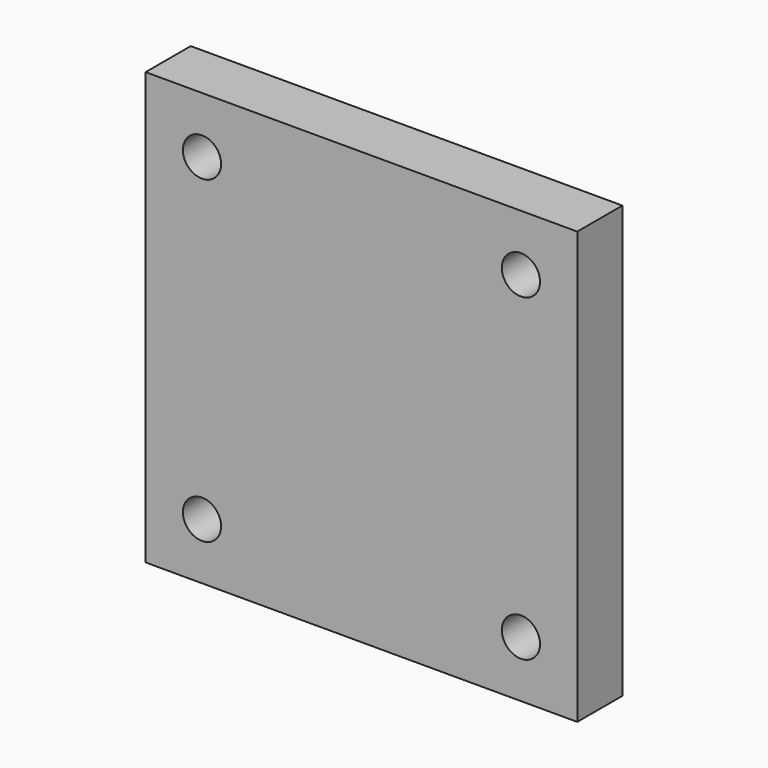
from build123d import *

# Parameters (mm, degrees)
F0_W     = 48.6210244843
F0_H     = 48.6210244843
F0_R     = 2.15265
F1_DEPTH = 6.35
F6_W     = 2.794
F6_H     = 1.27
F8_R     = 0.2032


with BuildPart() as f1:
    # F0 (on Front) → F1 (new body)
    with BuildSketch(Plane.XZ):
        Rectangle(F0_W, F0_H)
        with Locations((-17.9605122421, -17.9605122421)):
            Circle(F0_R, mode=Mode.SUBTRACT)
        with Locations((17.9605122421, -17.9605122421)):
            Circle(F0_R, mode=Mode.SUBTRACT)
        with Locations((-17.9605122421, 17.9605122421)):
            Circle(F0_R, mode=Mode.SUBTRACT)
        with Locations((17.9605122421, 17.9605122421)):
            Circle(F0_R, mode=Mode.SUBTRACT)
    extrude(amount=F1_DEPTH)

    # F6 (on 3pt) → F7 (revolve, cut)
    with BuildSketch(Plane(origin=(0, 0, 0), x_dir=(1, 0, 0), z_dir=(0, 0, -1))):
        with Locations((-19.7993, 0.635)):
            Rectangle(F6_W, F6_H)
    revolve(axis=Axis((0, 0.4501026124, 0), (0, -1, 0)), mode=Mode.SUBTRACT)

    # F8
    f8_edges = [f1.edges().sort_by_distance(p)[0] for p in [
        (21.1963, -1.27, 0),
        (18.4023, 0, 0),
    ]]
    fillet(f8_edges, radius=F8_R)


solid = f1.part
